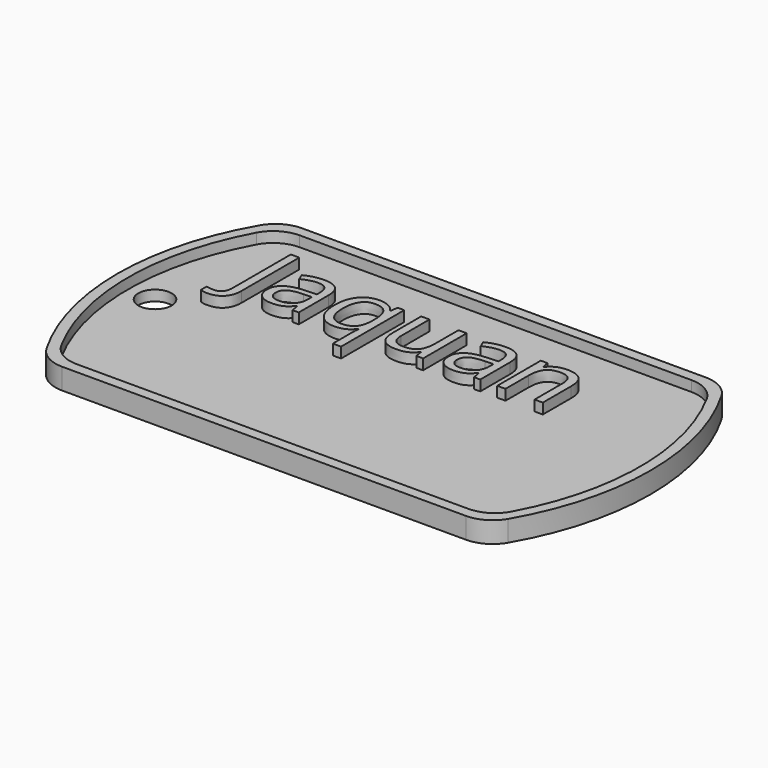
from build123d import *

# Parameters (mm, degrees)
F1_DEPTH     = 1
F3_DEPTH     = 1
F4_R         = 1.5875
F5_DEPTH     = 1
F6_TEXT_SIZE = 9.7016833024
F7_DEPTH     = 1


# Not quite as in the source:
# - Text() gives the source's letters only with a copy of the font that has no kerning and outlines rounded to 1/6400 em; it was checked with that copy


with BuildPart() as f1:
    # F0 (on Top) → F1 (new body)
    with BuildSketch(Plane.XY):
        with BuildLine():
            ThreePointArc((-19.2474145991, 14.2875), (-20.8349145991, 13.862130657), (-21.9970452561, 12.7))
            ThreePointArc((-21.9970452561, 12.7), (-25.4, 0), (-21.9970452561, -12.7))
            ThreePointArc((-21.9970452561, -12.7), (-20.8349145991, -13.862130657), (-19.2474145991, -14.2875))
            Line((-19.2474145991, -14.2875), (19.2474145991, -14.2875))
            ThreePointArc((19.2474145991, -14.2875), (20.8349145991, -13.862130657), (21.9970452561, -12.7))
            ThreePointArc((21.9970452561, -12.7), (25.4, 0), (21.9970452561, 12.7))
            ThreePointArc((21.9970452561, 12.7), (20.8349145991, 13.862130657), (19.2474145991, 14.2875))
            Line((19.2474145991, 14.2875), (-19.2474145991, 14.2875))
        make_face()
    extrude(amount=F1_DEPTH)

    # F2 (on face) → F3 (join)
    with BuildSketch(Plane.XY.offset(1)):
        with BuildLine():
            Line((19.2474145991, 14.2875), (-19.2474145991, 14.2875))
            ThreePointArc((-19.2474145991, 14.2875), (-20.8349145991, 13.862130657), (-21.9970452561, 12.7))
            ThreePointArc((-21.9970452561, 12.7), (-25.4, 0), (-21.9970452561, -12.7))
            ThreePointArc((-21.9970452561, -12.7), (-20.8349145991, -13.862130657), (-19.2474145991, -14.2875))
            Line((-19.2474145991, -14.2875), (19.2474145991, -14.2875))
            ThreePointArc((19.2474145991, -14.2875), (20.8349145991, -13.862130657), (21.9970452561, -12.7))
            ThreePointArc((21.9970452561, -12.7), (25.4, 0), (21.9970452561, 12.7))
            ThreePointArc((21.9970452561, 12.7), (20.8349145991, 13.862130657), (19.2474145991, 14.2875))
        make_face()
        with BuildLine():
            ThreePointArc((-21.4526124879, 11.6252061249), (-20.2856017842, 12.8404540819), (-18.6611352482, 13.2875))
            Line((-18.6611352482, 13.2875), (18.6611352482, 13.2875))
            ThreePointArc((18.6611352482, 13.2875), (20.2856017842, 12.8404540819), (21.4526124879, 11.6252061249))
            ThreePointArc((21.4526124879, 11.6252061249), (24.4, 0), (21.4526124879, -11.6252061249))
            ThreePointArc((21.4526124879, -11.6252061249), (20.2856017842, -12.8404540819), (18.6611352482, -13.2875))
            Line((18.6611352482, -13.2875), (-18.6611352482, -13.2875))
            ThreePointArc((-18.6611352482, -13.2875), (-20.2856017842, -12.8404540819), (-21.4526124879, -11.6252061249))
            ThreePointArc((-21.4526124879, -11.6252061249), (-24.4, 0), (-21.4526124879, 11.6252061249))
        make_face(mode=Mode.SUBTRACT)
    extrude(amount=F3_DEPTH)

    # F4 (on face) → F5 (cut)
    with BuildSketch(Plane.XY.offset(1)):
        with Locations((-21.821282804, 0)):
            Circle(F4_R)
    extrude(amount=-F5_DEPTH, mode=Mode.SUBTRACT)

    # F6 (on face) → F7 (join)
    with BuildSketch(Plane.XY.offset(1)):
        with Locations((-18.1550048292, 3.5402297508)):
            Text('Jaquan', F6_TEXT_SIZE, font='Open Sans', text_align=(TextAlign.LEFT, TextAlign.BOTTOM))
    extrude(amount=F7_DEPTH)


solid = f1.part
